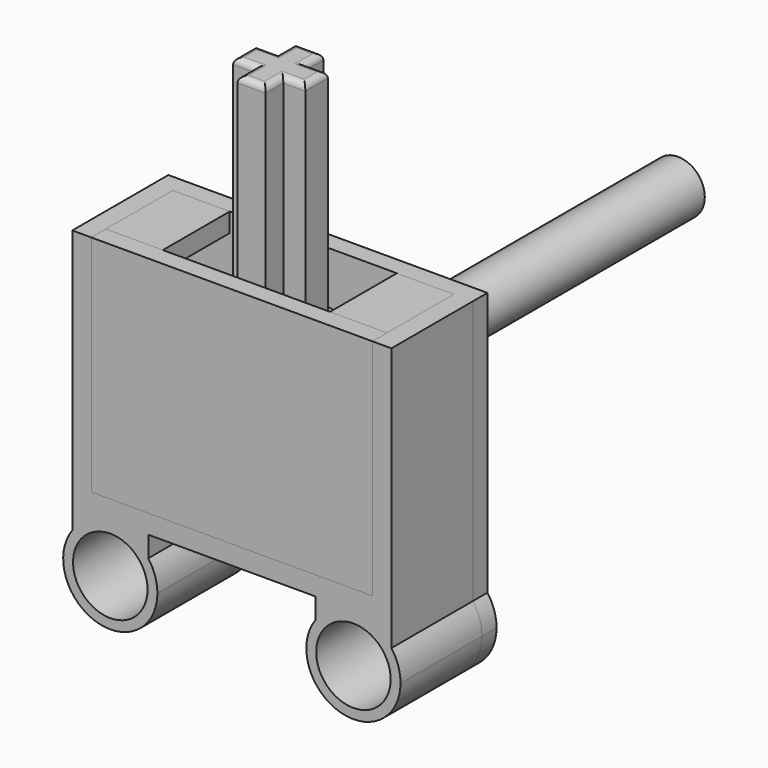
from build123d import *

# Parameters (mm, degrees)
F0_R      = 1.615
F0_R_2    = 1.35
F0_R_3    = 2.45
F0_R_4    = 1.315
F0_R_5    = 0.75
F0_R_6    = 1.015
F0_W      = 3.75
F0_H      = 1.25
F1_DEPTH  = 1.2
F2_DEPTH  = 6.7
F3_DEPTH  = 5.5
F4_DEPTH  = 5
F5_DEPTH  = 7
F8_R      = 0.725
F9_DEPTH  = 1.2
F10_DEPTH = 5.4
F11_DEPTH = 5.4
F14_DEPTH = 15
F15_R     = 0.4
F17_R     = 1.765
F17_R_2   = 1.615
F18_DEPTH = 20


# Not quite as in the source:
# - a fillet or chamfer that OpenCascade refuses, or shapes differently, is made with other operations: its cross-section is extruded or revolved along the edge and cut away or added


with BuildPart() as f1:
    # F0 (on Front) → F1 (new body)
    with BuildSketch(Plane.XZ):
        Polygon((0, 3.75), (-5.5, 3.75), (-9.25, 3.75), (-9.25, -9.75), (9.25, -9.75), (9.25, 3.75), (5.5, 3.75), align=None)
        with BuildLine():
            add(Edge.make_bspline(
                [(-6.5, -2.385), (-6.5, -9.3132032303), (3.25, -5.8491016151), (13, -2.385), (3.25, 1.0791016151), (-6.5, 4.5432032303), (-6.5, -2.385)],
                knots=[0, 0, 0, 2.0943951024, 2.0943951024, 4.1887902048, 4.1887902048, 6.2831853072, 6.2831853072, 6.2831853072], degree=2, weights=[1, 0.5, 1, 0.5, 1, 0.5, 1]))
        make_face(mode=Mode.SUBTRACT)
        with BuildLine():
            add(Edge.make_bspline(
                [(-6.5, -2.385), (-6.5, -9.3132032303), (3.25, -5.8491016151), (13, -2.385), (3.25, 1.0791016151), (-6.5, 4.5432032303), (-6.5, -2.385)],
                knots=[0, 0, 0, 2.0943951024, 2.0943951024, 4.1887902048, 4.1887902048, 6.2831853072, 6.2831853072, 6.2831853072], degree=2, weights=[1, 0.5, 1, 0.5, 1, 0.5, 1]))
        make_face()
        with Locations((-4, -1.9384471872)):
            Circle(F0_R, mode=Mode.SUBTRACT)
        with Locations((0, -4)):
            Circle(F0_R, mode=Mode.SUBTRACT)
        with Locations((4, -1.9384471872)):
            Circle(F0_R, mode=Mode.SUBTRACT)
        Circle(F0_R_2, mode=Mode.SUBTRACT)
        Polygon((-9.25, 3.75), (-9.25, 5), (-10.5, 5), (-10.5, -11), (-5.5, -11), (5.5, -11), (10.5, -11), (10.5, 5), (9.25, 5), (9.25, 3.75), (9.25, -9.75), (-9.25, -9.75), align=None)
        with BuildLine():
            ThreePointArc((-5.5, -12.366969722), (-8, -11.1), (-10.5, -12.366969722))
            ThreePointArc((-10.5, -12.366969722), (-8.9643650761, -17.1461839725), (-4.9, -14.2))
            ThreePointArc((-4.9, -14.2), (-5.0538160275, -13.2356349239), (-5.5, -12.366969722))
        make_face()
        with Locations((-8, -14.2)):
            Circle(F0_R_3, mode=Mode.SUBTRACT)
        with BuildLine():
            ThreePointArc((11.1, -14.2), (10.9461839725, -13.2356349239), (10.5, -12.366969722))
            ThreePointArc((10.5, -12.366969722), (8, -11.1), (5.5, -12.366969722))
            ThreePointArc((5.5, -12.366969722), (7.0356349239, -17.1461839725), (11.1, -14.2))
        make_face()
        with Locations((8, -14.2)):
            Circle(F0_R_3, mode=Mode.SUBTRACT)
        Polygon((5.5, 5), (0, 5), (-5.5, 5), (-5.5, 3.75), (0, 3.75), (5.5, 3.75), align=None)
        with Locations((-4, -1.9384471872)):
            Circle(F0_R)
        with Locations((-4, -1.9384471872)):
            Circle(F0_R_4, mode=Mode.SUBTRACT)
        with Locations((0, -4)):
            Circle(F0_R)
        with Locations((0, -4)):
            Circle(F0_R_4, mode=Mode.SUBTRACT)
        with Locations((4, -1.9384471872)):
            Circle(F0_R)
        with Locations((4, -1.9384471872)):
            Circle(F0_R_4, mode=Mode.SUBTRACT)
        Circle(F0_R_2)
        Circle(F0_R_5, mode=Mode.SUBTRACT)
        with Locations((4, -1.9384471872)):
            Circle(F0_R_4)
        with Locations((4, -1.9384471872)):
            Circle(F0_R_6, mode=Mode.SUBTRACT)
        with Locations((0, -4)):
            Circle(F0_R_4)
        with Locations((0, -4)):
            Circle(F0_R_6, mode=Mode.SUBTRACT)
        with Locations((-4, -1.9384471872)):
            Circle(F0_R_4)
        with Locations((-4, -1.9384471872)):
            Circle(F0_R_6, mode=Mode.SUBTRACT)
        with Locations((-7.375, 4.375)):
            Rectangle(F0_W, F0_H)
        with Locations((7.375, 4.375)):
            Rectangle(F0_W, F0_H)
        with BuildLine():
            Line((-5.5, -11), (-10.5, -11))
            Line((-10.5, -11), (-10.5, -12.366969722))
            ThreePointArc((-10.5, -12.366969722), (-8, -11.1), (-5.5, -12.366969722))
            Line((-5.5, -12.366969722), (-5.5, -11))
        make_face()
        with BuildLine():
            Line((10.5, -12.366969722), (10.5, -11))
            Line((10.5, -11), (5.5, -11))
            Line((5.5, -11), (5.5, -12.366969722))
            ThreePointArc((5.5, -12.366969722), (8, -11.1), (10.5, -12.366969722))
        make_face()
        Circle(F0_R_5)
    extrude(amount=-F1_DEPTH)

    # F0 (on Front) → F2 (join)
    with BuildSketch(Plane.XZ):
        Polygon((-9.25, 3.75), (-9.25, 5), (-10.5, 5), (-10.5, -11), (-5.5, -11), (5.5, -11), (10.5, -11), (10.5, 5), (9.25, 5), (9.25, 3.75), (9.25, -9.75), (-9.25, -9.75), align=None)
        with BuildLine():
            ThreePointArc((-5.5, -12.366969722), (-8, -11.1), (-10.5, -12.366969722))
            ThreePointArc((-10.5, -12.366969722), (-8.9643650761, -17.1461839725), (-4.9, -14.2))
            ThreePointArc((-4.9, -14.2), (-5.0538160275, -13.2356349239), (-5.5, -12.366969722))
        make_face()
        with Locations((-8, -14.2)):
            Circle(F0_R_3, mode=Mode.SUBTRACT)
        with BuildLine():
            Line((-5.5, -11), (-10.5, -11))
            Line((-10.5, -11), (-10.5, -12.366969722))
            ThreePointArc((-10.5, -12.366969722), (-8, -11.1), (-5.5, -12.366969722))
            Line((-5.5, -12.366969722), (-5.5, -11))
        make_face()
        with BuildLine():
            ThreePointArc((11.1, -14.2), (10.9461839725, -13.2356349239), (10.5, -12.366969722))
            ThreePointArc((10.5, -12.366969722), (8, -11.1), (5.5, -12.366969722))
            ThreePointArc((5.5, -12.366969722), (7.0356349239, -17.1461839725), (11.1, -14.2))
        make_face()
        with Locations((8, -14.2)):
            Circle(F0_R_3, mode=Mode.SUBTRACT)
        with BuildLine():
            Line((10.5, -12.366969722), (10.5, -11))
            Line((10.5, -11), (5.5, -11))
            Line((5.5, -11), (5.5, -12.366969722))
            ThreePointArc((5.5, -12.366969722), (8, -11.1), (10.5, -12.366969722))
        make_face()
    extrude(amount=F2_DEPTH)

    # F0 (on Front) → F3 (join)
    with BuildSketch(Plane.XZ):
        with Locations((-7.375, 4.375)):
            Rectangle(F0_W, F0_H)
        with Locations((7.375, 4.375)):
            Rectangle(F0_W, F0_H)
        Circle(F0_R_2)
        Circle(F0_R_5, mode=Mode.SUBTRACT)
    extrude(amount=F3_DEPTH)

    # F0 (on Front) → F4 (join)
    with BuildSketch(Plane.XZ):
        with Locations((-4, -1.9384471872)):
            Circle(F0_R)
        with Locations((-4, -1.9384471872)):
            Circle(F0_R_4, mode=Mode.SUBTRACT)
        with Locations((0, -4)):
            Circle(F0_R)
        with Locations((0, -4)):
            Circle(F0_R_4, mode=Mode.SUBTRACT)
        with Locations((4, -1.9384471872)):
            Circle(F0_R)
        with Locations((4, -1.9384471872)):
            Circle(F0_R_4, mode=Mode.SUBTRACT)
    extrude(amount=-F4_DEPTH)

    # F0 (on Front) → F5 (join)
    with BuildSketch(Plane.XZ):
        with Locations((-4, -1.9384471872)):
            Circle(F0_R_4)
        with Locations((-4, -1.9384471872)):
            Circle(F0_R_6, mode=Mode.SUBTRACT)
        with Locations((0, -4)):
            Circle(F0_R_4)
        with Locations((0, -4)):
            Circle(F0_R_6, mode=Mode.SUBTRACT)
        with Locations((4, -1.9384471872)):
            Circle(F0_R_4)
        with Locations((4, -1.9384471872)):
            Circle(F0_R_6, mode=Mode.SUBTRACT)
    extrude(amount=-F5_DEPTH)

    # F6: fillet of radius 0.5 on 3 edges, made by hand

    # F6_s1 → F6_t2 (revolve, cut)
    with BuildSketch(Plane.XY.offset(-1.9384471872)):
        with BuildLine():
            ThreePointArc((5.615, 4.5417424305), (5.5333300133, 4.8156037093), (5.315, 5))
            Line((5.315, 5), (5.615, 5))
            Line((5.615, 5), (5.615, 4.5417424305))
        make_face()
    revolve(axis=Axis((4, 5, -1.9384471872), (0, -1, 0)), mode=Mode.SUBTRACT)

    # F6_s3 → F6_t4 (revolve, cut)
    with BuildSketch(Plane.XY.offset(-4)):
        with BuildLine():
            ThreePointArc((1.615, 4.5417424305), (1.5333300133, 4.8156037093), (1.315, 5))
            Line((1.315, 5), (1.615, 5))
            Line((1.615, 5), (1.615, 4.5417424305))
        make_face()
    revolve(axis=Axis((0, 5, -4), (0, -1, 0)), mode=Mode.SUBTRACT)

    # F6_s5 → F6_t6 (revolve, cut)
    with BuildSketch(Plane.XY.offset(-1.9384471872)):
        with BuildLine():
            ThreePointArc((-2.385, 4.5417424305), (-2.4666699867, 4.8156037093), (-2.685, 5))
            Line((-2.685, 5), (-2.385, 5))
            Line((-2.385, 5), (-2.385, 4.5417424305))
        make_face()
    revolve(axis=Axis((-4, 5, -1.9384471872), (0, -1, 0)), mode=Mode.SUBTRACT)

    # F7: fillet of radius 0.5 on 3 edges, made by hand

    # F7_s1 → F7_t2 (revolve, cut)
    with BuildSketch(Plane.XY.offset(-1.9384471872)):
        with BuildLine():
            ThreePointArc((5.315, 6.5417424305), (5.2333300133, 6.8156037093), (5.015, 7))
            Line((5.015, 7), (5.315, 7))
            Line((5.315, 7), (5.315, 6.5417424305))
        make_face()
    revolve(axis=Axis((4, 7, -1.9384471872), (0, -1, 0)), mode=Mode.SUBTRACT)

    # F7_s3 → F7_t4 (revolve, cut)
    with BuildSketch(Plane.XY.offset(-4)):
        with BuildLine():
            ThreePointArc((1.315, 6.5417424305), (1.2333300133, 6.8156037093), (1.015, 7))
            Line((1.015, 7), (1.315, 7))
            Line((1.315, 7), (1.315, 6.5417424305))
        make_face()
    revolve(axis=Axis((0, 7, -4), (0, -1, 0)), mode=Mode.SUBTRACT)

    # F7_s5 → F7_t6 (revolve, cut)
    with BuildSketch(Plane.XY.offset(-1.9384471872)):
        with BuildLine():
            ThreePointArc((-2.685, 6.5417424305), (-2.7666699867, 6.8156037093), (-2.985, 7))
            Line((-2.985, 7), (-2.685, 7))
            Line((-2.685, 7), (-2.685, 6.5417424305))
        make_face()
    revolve(axis=Axis((-4, 7, -1.9384471872), (0, -1, 0)), mode=Mode.SUBTRACT)


with BuildPart() as f9:
    # F8 (on face) → F9 (new body)
    with BuildSketch(Plane.XZ.offset(5.5)):
        Polygon((-5.5, 5), (-9.25, 5), (-9.25, -9.75), (9.25, -9.75), (9.25, 5), (5.5, 5), align=None)
        Circle(F8_R, mode=Mode.SUBTRACT)
        Circle(F8_R)
    extrude(amount=F9_DEPTH)

    # F8 (on face) → F10 (join)
    with BuildSketch(Plane.XZ.offset(5.5)):
        Circle(F8_R)
    extrude(amount=-F10_DEPTH)


with BuildPart() as f11:
    # F0 (on Front) → F11 (new body)
    with BuildSketch(Plane.XZ):
        with BuildLine():
            add(Edge.make_bspline(
                [(-6.5, -2.385), (-6.5, -9.3132032303), (3.25, -5.8491016151), (13, -2.385), (3.25, 1.0791016151), (-6.5, 4.5432032303), (-6.5, -2.385)],
                knots=[0, 0, 0, 2.0943951024, 2.0943951024, 4.1887902048, 4.1887902048, 6.2831853072, 6.2831853072, 6.2831853072], degree=2, weights=[1, 0.5, 1, 0.5, 1, 0.5, 1]))
        make_face()
        with Locations((-4, -1.9384471872)):
            Circle(F0_R, mode=Mode.SUBTRACT)
        with Locations((0, -4)):
            Circle(F0_R, mode=Mode.SUBTRACT)
        with Locations((4, -1.9384471872)):
            Circle(F0_R, mode=Mode.SUBTRACT)
        Circle(F0_R_2, mode=Mode.SUBTRACT)
        with Locations((-4, -1.9384471872)):
            Circle(F0_R)
        with Locations((-4, -1.9384471872)):
            Circle(F0_R_4, mode=Mode.SUBTRACT)
        with Locations((-4, -1.9384471872)):
            Circle(F0_R_4)
        with Locations((-4, -1.9384471872)):
            Circle(F0_R_6, mode=Mode.SUBTRACT)
        with Locations((-4, -1.9384471872)):
            Circle(F0_R_6)
        with Locations((0, -4)):
            Circle(F0_R)
        with Locations((0, -4)):
            Circle(F0_R_4, mode=Mode.SUBTRACT)
        with Locations((0, -4)):
            Circle(F0_R_4)
        with Locations((0, -4)):
            Circle(F0_R_6, mode=Mode.SUBTRACT)
        with Locations((0, -4)):
            Circle(F0_R_6)
        with Locations((4, -1.9384471872)):
            Circle(F0_R)
        with Locations((4, -1.9384471872)):
            Circle(F0_R_4, mode=Mode.SUBTRACT)
        with Locations((4, -1.9384471872)):
            Circle(F0_R_4)
        with Locations((4, -1.9384471872)):
            Circle(F0_R_6, mode=Mode.SUBTRACT)
        with Locations((4, -1.9384471872)):
            Circle(F0_R_6)
    extrude(amount=F11_DEPTH)

    # F13 (on offset) → F14 (join)
    with BuildSketch(Plane.XY.offset(1.4)):
        Polygon((0.925, -0.325), (0, -0.325), (-0.925, -0.325), (-0.925, -1.775), (-2.375, -1.775), (-2.375, -2.7), (-2.375, -3.625), (-0.925, -3.625), (-0.925, -5.075), (0, -5.075), (0.925, -5.075), (0.925, -3.625), (2.375, -3.625), (2.375, -2.7), (2.375, -1.775), (0.925, -1.775), align=None)
    extrude(amount=F14_DEPTH)

    # F15
    f15_edges = [f11.edges().sort_by_distance(p)[0] for p in [
        (0, -0.325, 16.4),
        (-0.925, -1.05, 16.4),
        (-1.65, -1.775, 16.4),
        (-2.375, -2.7, 16.4),
        (-1.65, -3.625, 16.4),
        (-0.925, -4.35, 16.4),
        (0, -5.075, 16.4),
        (0.925, -4.35, 16.4),
        (1.65, -3.625, 16.4),
        (2.375, -2.7, 16.4),
        (1.65, -1.775, 16.4),
        (0.925, -1.05, 16.4),
    ]]
    fillet(f15_edges, radius=F15_R)


with BuildPart() as f18:
    # F17 (on offset) → F18 (new body)
    with BuildSketch(Plane.XZ.offset(-10)):
        with Locations((0, -4)):
            Circle(F17_R)
        with Locations((0, -4)):
            Circle(F17_R_2, mode=Mode.SUBTRACT)
    extrude(amount=-F18_DEPTH)


solid = Compound([f1.part, f9.part, f11.part, f18.part])
